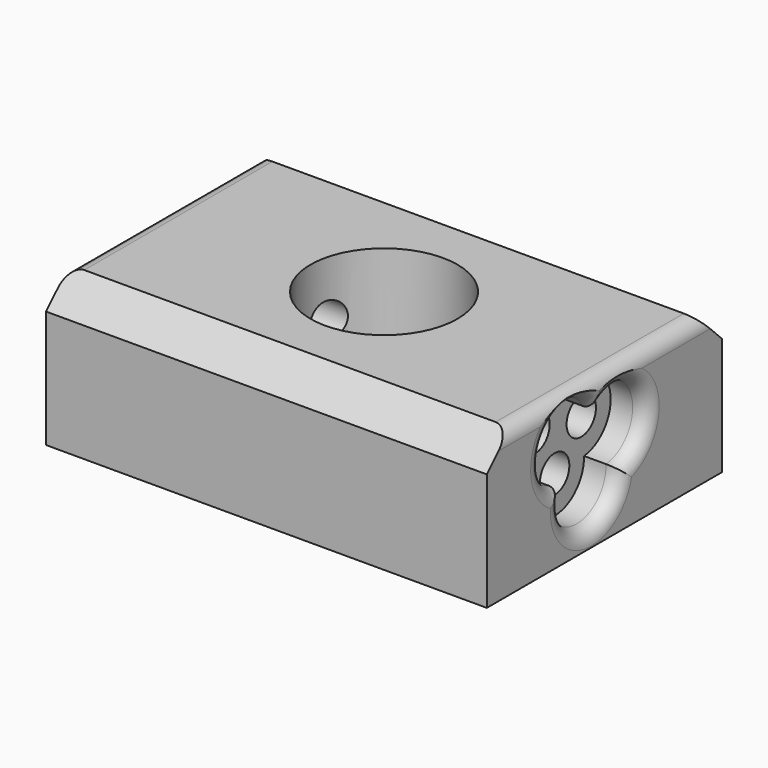
from build123d import *

# Parameters (mm, degrees)
F0_W           = 76.2
F0_H           = 50.8
F0_R           = 12.7
F1_DEPTH       = 25.4
F3_D           = 6.35
F3_CBORE_D     = 12.7
F3_CBORE_DEPTH = 6.35
F4_SIZE        = 5.08
F5_R           = 2.54
F6_T1_DEPTH    = 53.34
F6_T4_ANGLE    = 333.5496050311
F6_T6_ANGLE    = 313.8522207809
F6_T8_ANGLE    = 339.5771348814


# Not quite as in the source:
# - a fillet or chamfer that OpenCascade refuses, or shapes differently, is made with other operations: its cross-section is extruded or revolved along the edge and cut away or added


with BuildPart() as f1:
    # F0 (on Top) → F1 (new body)
    with BuildSketch(Plane.XY):
        Rectangle(F0_W, F0_H)
        Circle(F0_R, mode=Mode.SUBTRACT)
    extrude(amount=F1_DEPTH)

    # F3 (through all)
    with Locations(Plane.YZ.offset(38.1)):
        with Locations((-7.0466324687, 17.1319264919), (2.941543702, 15.6153971329), (-2.8108085971, 9.1309268028)):
            CounterBoreHole(F3_D / 2, F3_CBORE_D / 2, F3_CBORE_DEPTH)

    # F4
    f4_edges = [f1.edges().sort_by_distance(p)[0] for p in [
        (0, -25.4, 25.4),
        (0, 25.4, 25.4),
    ]]
    chamfer(f4_edges, length=F4_SIZE)

    # F5
    f5_edges = [f1.edges().sort_by_distance(p)[0] for p in [
        (-38.1, 0, 25.4),
    ]]
    fillet(f5_edges, radius=F5_R)

    # F6: fillet of radius 2.54 on 4 edges, made by hand

    # F6_s2 → F6_t1 (cut)
    with BuildSketch(Plane.XZ.offset(-26.67)):
        with BuildLine():
            ThreePointArc((35.56, 25.4), (37.3560512242, 24.6560512242), (38.1, 22.86))
            Line((38.1, 22.86), (38.1, 25.4))
            Line((38.1, 25.4), (35.56, 25.4))
        make_face()
    extrude(amount=F6_T1_DEPTH, mode=Mode.SUBTRACT)

    # F6_s3 → F6_t4 (revolve, cut)
    with BuildSketch(Plane(origin=(0, -6.4599960512, 8.2833530872), x_dir=(1, 0, 0), z_dir=(0, -0.6149714639, 0.7885493634))):
        with BuildLine():
            ThreePointArc((38.1, 3.032576048), (37.3560512242, 4.8286272723), (35.56, 5.572576048))
            Line((35.56, 5.572576048), (38.1, 5.572576048))
            Line((38.1, 5.572576048), (38.1, 3.032576048))
        make_face()
    revolve(axis=Axis((38.1, 2.941543702, 15.6153971329), (1, 0, 0)), revolution_arc=F6_T4_ANGLE, mode=Mode.SUBTRACT)

    # F6_s5 → F6_t6 (revolve, cut)
    with BuildSketch(Plane(origin=(0, -0.3361656341, -0.0902154954), x_dir=(1, 0, 0), z_dir=(0, 0.9658250629, 0.2591948067))):
        with BuildLine():
            ThreePointArc((38.1, -18.4374249449), (37.3560512242, -16.6413737207), (35.56, -15.8974249449))
            Line((35.56, -15.8974249449), (38.1, -15.8974249449))
            Line((38.1, -15.8974249449), (38.1, -18.4374249449))
        make_face()
    revolve(axis=Axis((38.1, -2.8108085971, 9.1309268028), (1, 0, 0)), revolution_arc=F6_T6_ANGLE, mode=Mode.SUBTRACT)

    # F6_s7 → F6_t8 (revolve, cut)
    with BuildSketch(Plane(origin=(0, 5.5955772378, 10.1893133195), x_dir=(1, 0, 0), z_dir=(0, -0.4813542865, -0.8765261267))):
        with BuildLine():
            ThreePointArc((38.1, 5.5330837175), (37.3560512242, 7.3291349418), (35.56, 8.0730837175))
            Line((35.56, 8.0730837175), (38.1, 8.0730837175))
            Line((38.1, 8.0730837175), (38.1, 5.5330837175))
        make_face()
    revolve(axis=Axis((38.1, -7.0466324687, 17.1319264919), (1, 0, 0)), revolution_arc=F6_T8_ANGLE, mode=Mode.SUBTRACT)


solid = f1.part
